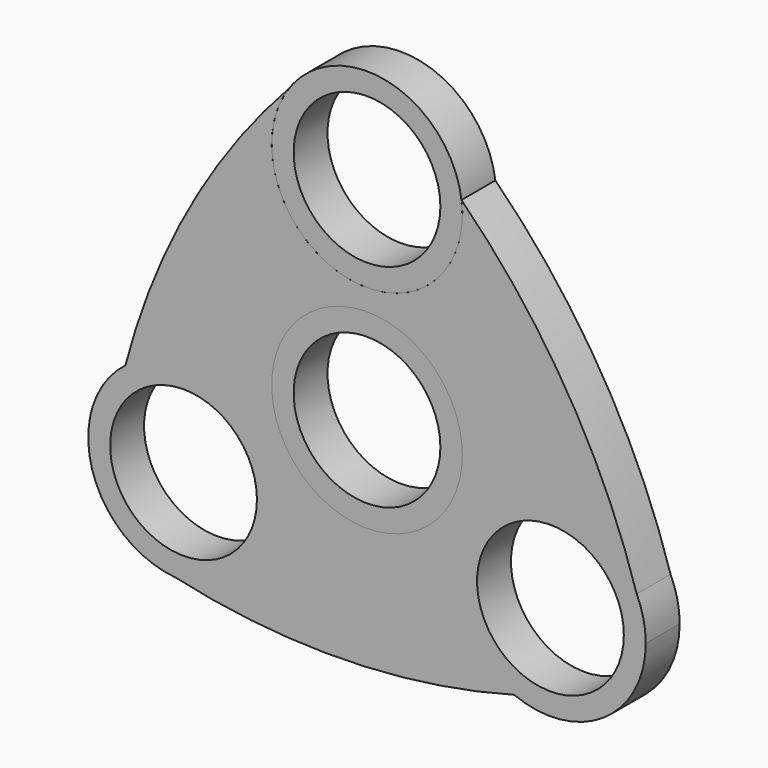
from build123d import *

# Parameters (mm, degrees)
F0_R     = 14.2875
F0_R_2   = 10.9982
F2_DEPTH = 6.35
F1_R     = 10.9982
F1_R_2   = 14.2875


with BuildPart() as f2:
    # F0 (on Front) → F2 (new body)
    with BuildSketch(Plane.XZ):
        with Locations((0, 31.75)):
            Circle(F0_R)
        with Locations((0, 31.75)):
            Circle(F0_R_2, mode=Mode.SUBTRACT)
    extrude(amount=F2_DEPTH)


with BuildPart() as f2b:
    # F0 (on Front) → F2, piece 2 (new body)
    with BuildSketch(Plane.XZ):
        Circle(F0_R)
        Circle(F0_R_2, mode=Mode.SUBTRACT)
    extrude(amount=F2_DEPTH)


with BuildPart() as f2c:
    # F1 (on face) → F2, piece 3 (new body)
    with BuildSketch(Plane.XZ):
        with BuildLine():
            ThreePointArc((41.7838065702, -15.875), (41.4405176602, -12.7618611777), (40.4271474867, -9.7983224999))
            ThreePointArc((40.4271474867, -9.7983224999), (17.1515631107, -6.0201058347), (22.0535595667, -29.0851915696))
            ThreePointArc((22.0535595667, -29.0851915696), (35.4451872599, -27.7471502699), (41.7838065702, -15.875))
        make_face()
        with Locations((27.4963065702, -15.875)):
            Circle(F1_R, mode=Mode.SUBTRACT)
        with BuildLine():
            ThreePointArc((-13.2088065702, -15.875), (-21.1891631837, -3.0549922561), (-36.2152945566, -4.5563470438))
            ThreePointArc((-36.2152945566, -4.5563470438), (-41.2032669986, -19.9063635489), (-28.6991699428, -30.1117754761))
            ThreePointArc((-28.6991699428, -30.1117754761), (-17.8281437195, -26.3944716285), (-13.2088065702, -15.875))
        make_face()
        with Locations((-27.4963065702, -15.875)):
            Circle(F1_R, mode=Mode.SUBTRACT)
        with BuildLine():
            ThreePointArc((14.1617349899, 33.6415386135), (14.2560240761, 32.697857474), (14.2875, 31.75))
            ThreePointArc((14.2875, 31.75), (-4.2760482393, 18.1173895491), (-11.727977544, 39.910097976))
            ThreePointArc((-11.727977544, 39.910097976), (-26.7194199084, 19.1900581454), (-36.2152945566, -4.5563470438))
            ThreePointArc((-36.2152945566, -4.5563470438), (-21.1891631837, -3.0549922561), (-13.2088065702, -15.875))
            ThreePointArc((-13.2088065702, -15.875), (-17.8281437195, -26.3944716285), (-28.6991699428, -30.1117754761))
            ThreePointArc((-28.6991699428, -30.1117754761), (-3.2593678998, -32.7347254878), (22.0535595667, -29.0851915696))
            ThreePointArc((22.0535595667, -29.0851915696), (17.1515631107, -6.0201058347), (40.4271474867, -9.7983224999))
            ThreePointArc((40.4271474867, -9.7983224999), (29.9787878083, 13.5446673424), (14.1617349899, 33.6415386135))
        make_face()
        Circle(F1_R_2, mode=Mode.SUBTRACT)
    extrude(amount=F2_DEPTH)


solid = Compound([f2.part, f2b.part, f2c.part])
